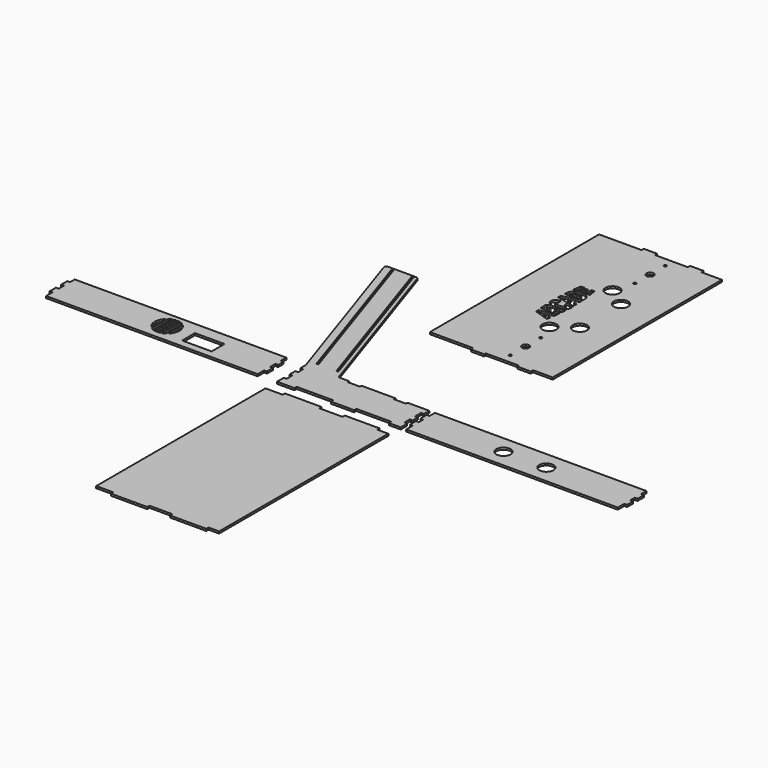
from build123d import *

# Parameters (mm, degrees)
F1_DEPTH = 4.45
F0_R     = 3
F0_R_2   = 8.087272744
F0_R_3   = 16.129
F0_W     = 66.7005181313
F0_H     = 36.3053381443


# Not quite as in the source:
# - ends of sketch curves that miss each other by under 0.0002 mm in the source are joined
# - a feature names something its author has since deleted; it is built from what else it names


with BuildPart() as f1:
    # F0 (on Top) → F1 (new body)
    with BuildSketch(Plane.XY):
        with BuildLine():
            Line((-13.1345508408, -164.6919741164), (-133.2231766972, 195.5739079059))
            ThreePointArc((-133.2231766972, 195.5739079059), (-135.0430417624, 198.0489800139), (-137.9665931933, 198.9927690934))
            Line((-137.9665931933, 198.9927690934), (-188.0199429035, 198.9927690934))
            Line((-188.0199429035, 198.9927690934), (-201.6566259516, 198.9927690934))
            ThreePointArc((-201.6566259516, 198.9927690934), (-205.7128368721, 196.9163205243), (-206.4000424478, 192.4116302809))
            Line((-206.4000424478, 192.4116302809), (-83.9924133672, -174.8112615001))
            Line((-83.9924133672, -174.8112615001), (-80.8544035681, -184.2252910137))
            Line((-80.8544035681, -184.2252910137), (-80.3456279762, -184.2252910137))
            Line((-80.3456279762, -184.2252910137), (-80.3456279762, -185.5896489572))
            Line((-80.3456279762, -185.5896489572), (-80.3456279762, -185.7516178083))
            Line((-80.3456279762, -185.7516178083), (-80.3456279762, -200.8809216976))
            Line((-80.3456279762, -200.8809216976), (-74.0156279762, -200.8809216976))
            Line((-74.0156279762, -200.8809216976), (-74.0156279762, -215.4068326941))
            Line((-74.0156279762, -215.4068326941), (-80.3456279762, -215.4068326941))
            Line((-80.3456279762, -215.4068326941), (-80.3456279762, -231.2078326941))
            Line((-80.3456279762, -231.2078326941), (-74.0156279762, -231.2078326941))
            Line((-74.0156279762, -231.2078326941), (-74.0156279762, -247.7338326941))
            Line((-74.0156279762, -247.7338326941), (-75.8956279762, -247.7338326941))
            Line((-75.8956279762, -247.7338326941), (-80.3456279762, -247.7338326941))
            Line((-80.3456279762, -247.7338326941), (-80.3456279762, -248.4956532717))
            Line((-80.3456279762, -248.4956532717), (-80.3456279762, -248.7336844206))
            Line((-80.3456279762, -248.7336844206), (-80.3456279762, -266.7746841908))
            Line((-80.3456279762, -266.7746841908), (-40.9429369935, -266.7746841908))
            Line((-40.9429369935, -266.7746841908), (-40.9429369935, -260.4446841907))
            Line((-40.9429369935, -260.4446841907), (41.3429330065, -260.4446841907))
            Line((41.3429330065, -260.4446841907), (41.3429330065, -266.7746841907))
            Line((41.3429330065, -266.7746841907), (93.9730530065, -266.7746841908))
            Line((93.9730530065, -266.7746841908), (93.9730530065, -260.4446841907))
            Line((93.9730530065, -260.4446841907), (172.7589230065, -260.4446841907))
            Line((172.7589230065, -260.4446841907), (172.7589230065, -266.7746841907))
            Line((172.7589230065, -266.7746841907), (199.3356065321, -266.7746841908))
            Line((199.3356065321, -266.7746841908), (199.3356065321, -248.4956532717))
            Line((199.3356065321, -248.4956532717), (193.0056065321, -248.4956532717))
            Line((193.0056065321, -248.4956532717), (193.0056065321, -232.9698022752))
            Line((193.0056065321, -232.9698022752), (199.3356065321, -232.9698022752))
            Line((199.3356065321, -232.9698022752), (199.3356065321, -218.5687422752))
            Line((199.3356065321, -218.5687422752), (193.0056065321, -218.5687422752))
            Line((193.0056065321, -218.5687422752), (193.0056065321, -201.0428905487))
            Line((193.0056065321, -201.0428905487), (199.3356065321, -201.0428905487))
            Line((199.3356065321, -201.0428905487), (199.3356065321, -185.7516178083))
            Line((199.3356065321, -185.7516178083), (149.9814315498, -185.7516178083))
            Line((149.9814315498, -185.7516178083), (149.9876286626, -190.2016178083))
            Line((149.9876286626, -190.2016178083), (122.5876286626, -190.2016178083))
            Line((122.5876286626, -190.2016178083), (122.5814315498, -185.7516178083))
            Line((122.5814315498, -185.7516178083), (45.8255372941, -185.7516178083))
            Line((45.8255372941, -185.7516178083), (45.8255372941, -190.2016178083))
            Line((45.8255372941, -190.2016178083), (18.4255372941, -190.2016178083))
            Line((18.4255372941, -190.2016178083), (17.9193401814, -185.7516178083))
            Line((17.9193401814, -185.7516178083), (-2.5108735826, -185.7516178083))
            ThreePointArc((-2.5108735826, -185.7516178083), (-5.4344250134, -184.8078287287), (-7.2542900787, -182.3327566208))
            Line((-7.2542900787, -182.3327566208), (-13.1345508408, -164.6919741164))
        make_face()
        Polygon((-68.8909804744, -169.5191176128), (-129.5292109794, 12.3955761507), (-190.322441274, 194.7752692889), (-185.872441274, 194.7752692889), (-125.1567108742, 12.6280758381), (-125.0792109794, 12.3955761507), (-64.4409804744, -169.5191176128), align=None, mode=Mode.SUBTRACT)
        Polygon((-145.372441274, 194.7752760296), (-140.922441274, 194.7752760296), (-19.4909804744, -169.5191108722), (-23.9409804744, -169.5191108722), (-84.6567108742, 12.6280825787), align=None, mode=Mode.SUBTRACT)
    extrude(amount=F1_DEPTH)


with BuildPart() as f1b:
    # F0 (on Top) → F1, piece 2 (new body)
    with BuildSketch(Plane.XY):
        Polygon((109.6645991251, 49.936733744), (109.6645991251, 43.606733744), (140.0583991251, 43.606733744), (140.0583991251, 48.056733744), (214.8266904935, 48.056733744), (214.8266904935, 43.606733744), (245.2266904935, 43.606733744), (245.2266904935, 49.936733744), (289.7008654758, 49.936733744), (289.7008654758, 528.386733744), (243.2266908545, 528.386733744), (243.2266908545, 534.716733744), (212.8266908545, 534.716733744), (212.8266908545, 528.386733744), (138.0584023733, 528.386733744), (138.0584023733, 534.716733744), (107.6646023733, 534.716733744), (107.6646023733, 528.386733744), (86.1305896078, 528.386733744), (11.8996296078, 528.386733744), (11.8996296078, 49.936733744), (86.1305896078, 49.936733744), align=None)
        with Locations((178.3758481905, 69.173247926)):
            Circle(F0_R, mode=Mode.SUBTRACT)
        with Locations((178.3758481905, 112.373247926)):
            Circle(F0_R_2, mode=Mode.SUBTRACT)
        with Locations((178.3758481905, 155.573247926)):
            Circle(F0_R, mode=Mode.SUBTRACT)
        with Locations((164.4027125835, 197.3344986652)):
            Circle(F0_R_3, mode=Mode.SUBTRACT)
        Polygon((144.38024237, 234.2502108202), (142.1130604967, 234.2502108202), (138.3344314918, 233.0626404271), (137.7946220263, 226.9088669107), (141.0334490165, 226.3150817141), (143.4625692591, 226.3150817141), (141.843155764, 218.1914640949), (140.1157833561, 218.9197583482), (134.9876381382, 220.3772260234), (123.0039752945, 224.2638251171), (109.6707962379, 228.5822598622), (108.9690484032, 235.0599175677), (128.5639636144, 238.406707196), (142.6528625115, 241.9694183752), (145.8329220252, 241.9694183752), align=None, mode=Mode.SUBTRACT)
        with BuildLine():
            add(Edge.make_bspline(
                [(128.5639636168, 260.5926792261), (126.6851334747, 261.6323850443), (125.1709058254, 262.4309195257), (123.2035912523, 262.8997626838)],
                knots=[0, 0, 0, 0, 0.1162972911, 0.1162972911, 0.1162972911, 0.1162972911], degree=3))
            add(Edge.make_bspline(
                [(131.0810425796, 258.8106178703), (130.4885197933, 259.5182474814), (129.4826550141, 260.0842943704), (128.5639636168, 260.5926792261)],
                knots=[0.9431341245, 0.9431341245, 0.9431341245, 0.9431341245, 1, 1, 1, 1], degree=3))
            Line((131.0810425796, 258.8106178703), (147.2951849037, 264.5332548154))
            Line((147.2951849037, 264.5332548154), (146.6391187302, 255.3441180101))
            Line((146.6391187302, 255.3441180101), (145.0819902192, 255.0326926987))
            Line((145.0819902192, 255.0326926987), (132.7204562794, 250.509393456))
            Line((132.7204562794, 250.509393456), (145.9027750667, 250.509393456))
            Line((145.9027750667, 250.509393456), (145.6217922195, 242.5632035718))
            Line((145.6217922195, 242.5632035718), (107.8536775567, 243.898710594))
            add(Edge.make_bspline(
                [(107.457601274, 243.9127161291), (107.5681389055, 243.8955344904), (107.7007268333, 243.8910975861), (107.8536775567, 243.898710594)],
                knots=[0.6431910445, 0.6431910445, 0.6431910445, 0.6431910445, 0.6525586544, 0.6525586544, 0.6525586544, 0.6525586544], degree=3))
            add(Edge.make_bspline(
                [(123.2035912523, 262.8997626838), (120.8214160248, 263.467473904), (114.6447375539, 263.6384105597), (104.4496833821, 259.1667517285), (108.5099601756, 247.3009629552), (106.515459915, 244.0591597631), (107.457601274, 243.9127161291)],
                knots=[0.1162972911, 0.1162972911, 0.1162972911, 0.1162972911, 0.2571189623, 0.4018084692, 0.5633484367, 0.6431910445, 0.6431910445, 0.6431910445, 0.6431910445], degree=3))
        make_face(mode=Mode.SUBTRACT)
        with BuildLine():
            add(Edge.make_bspline(
                [(118.4096939812, 278.2062657301), (118.008613675, 277.7544534713), (116.5254907196, 278.3846987718), (114.6860986223, 277.3704216428), (114.3121353636, 275.4818719009), (115.8822495107, 273.5639671058), (122.1543701521, 271.8085591307), (128.3372312156, 271.631565814), (134.6144229239, 272.2452065368), (138.281513843, 274.0041420395), (138.8901224926, 277.3280303811), (135.816879855, 277.8372704412), (132.3043819598, 278.6943910776), (132.8801296382, 279.7199041248), (133.0335295094, 286.4615207561), (131.517785638, 288.8097379759), (143.3081485383, 285.6706131454), (143.2876661042, 285.1920333687), (149.7203259126, 281.8270369122), (148.695702836, 273.0090093242), (145.8257996198, 267.8254041605), (137.5916580466, 263.7489152162), (126.7832057192, 262.9795878345), (114.9700731672, 264.1210882589), (108.486783454, 268.147637912), (104.5049371001, 272.096645925), (104.3359645468, 276.9661032929), (105.5397960824, 282.3849948376), (111.6880120097, 286.3382367425), (116.9904636561, 287.4430295691), (118.7674772932, 287.8835911533), (118.4200692992, 285.1487585296), (119.1960011795, 279.0920315629), (118.4096939812, 278.2062657301)],
                knots=[0, 0, 0, 0, 0.020494547, 0.0414693591, 0.0607350939, 0.0828404788, 0.1209521426, 0.159932456, 0.1980232824, 0.2276772762, 0.2510011815, 0.2764947931, 0.3037065377, 0.3173900946, 0.3574312462, 0.3741991924, 0.4232910827, 0.4368372532, 0.4735096835, 0.516799885, 0.5533151147, 0.5976483724, 0.648419728, 0.7005614172, 0.7421530316, 0.776720808, 0.8090959926, 0.8438514827, 0.8845213381, 0.9201032118, 0.9362852602, 0.9598209895, 1, 1, 1, 1], degree=3))
        make_face(mode=Mode.SUBTRACT)
        Polygon((146.2362490544, 313.2235731122), (146.9237737307, 313.160742366), (146.9237737307, 304.04164336), (144.6443654547, 304.04164336), (140.3559751758, 303.0352617738), (140.3559751758, 296.2421939832), (145.2770911107, 294.9842183974), (147.5267268667, 294.9842183974), (147.5016705642, 285.6739075454), (105.6019298682, 295.4861174461), (105.6019298682, 302.4049817708), align=None, mode=Mode.SUBTRACT)
        with BuildLine():
            ThreePointArc((107.1513079057, 320.8409628955), (125.426885077, 335.327875154), (146.2362490544, 324.7999257532))
            Line((146.2362490544, 324.7999257532), (146.9237737307, 313.6994063047))
            Line((146.9237737307, 313.6994063047), (106.4939506302, 312.5978863922))
            Line((106.4939506302, 312.5978863922), (107.1513079057, 320.8409628955))
        make_face(mode=Mode.SUBTRACT)
        Polygon((130.0334616295, 350.7802296276), (131.2729376142, 342.1865778554), (135.6725178609, 342.8211362717), (134.1524355063, 353.3603145865), (141.6923932681, 353.3603145865), (143.9817920473, 337.2012575192), (108.2818875652, 334.854008616), (111.446634675, 352.6165901807), (119.4676615248, 353.1822159079), (117.2535054335, 341.9162227896), (122.8425063143, 341.9162227896), (122.8425063143, 350.7802296276), align=None, mode=Mode.SUBTRACT)
        with Locations((208.4719767734, 228.5822598622)):
            Circle(F0_R_3, mode=Mode.SUBTRACT)
        with Locations((208.4719767734, 344.6277944729)):
            Circle(F0_R_3, mode=Mode.SUBTRACT)
        with Locations((164.4027125835, 375.8755556698)):
            Circle(F0_R_3, mode=Mode.SUBTRACT)
        with Locations((178.3758481905, 421.2868064091)):
            Circle(F0_R, mode=Mode.SUBTRACT)
        with Locations((178.3758481905, 464.4868064091)):
            Circle(F0_R_2, mode=Mode.SUBTRACT)
        with Locations((178.3758481905, 507.6868064091)):
            Circle(F0_R, mode=Mode.SUBTRACT)
        with BuildLine():
            Line((128.5639636168, 260.5926792261), (130.7771585832, 258.7033647236))
            Line((130.7771585832, 258.7033647236), (131.0810425796, 258.8106178703))
            add(Edge.make_bspline(
                [(131.0810425796, 258.8106178703), (130.4885197933, 259.5182474814), (129.4826550141, 260.0842943704), (128.5639636168, 260.5926792261)],
                knots=[0.9431341245, 0.9431341245, 0.9431341245, 0.9431341245, 1, 1, 1, 1], degree=3))
        make_face()
    extrude(amount=F1_DEPTH)


with BuildPart() as f1c:
    # F0 (on Top) → F1, piece 3 (new body)
    with BuildSketch(Plane.XY):
        Polygon((121.6972161211, 253.4000544932), (120.1217256436, 254.4976013836), (118.3763080916, 254.3745182559), (117.2535054335, 254.0755802312), (116.3434170136, 253.4000544932), (115.9999452481, 250.6342387882), (121.6972161211, 250.4327792945), align=None)
    extrude(amount=F1_DEPTH)


with BuildPart() as f1d:
    # F0 (on Top) → F1, piece 4 (new body)
    with BuildSketch(Plane.XY):
        Polygon((125.6387986193, 230.2756949452), (129.8662058959, 228.9461760905), (129.8662058959, 231.1009175268), align=None)
    extrude(amount=F1_DEPTH)


with BuildPart() as f1e:
    # F0 (on Top) → F1, piece 5 (new body)
    with BuildSketch(Plane.XY):
        Polygon((130.8137707362, 300.8135954973), (125.054859365, 299.5041205671), (130.8137707362, 298.1946465683), align=None)
    extrude(amount=F1_DEPTH)


with BuildPart() as f1f:
    # F0 (on Top) → F1, piece 6 (new body)
    with BuildSketch(Plane.XY):
        with BuildLine():
            Line((117.2535054335, 321.2757527021), (135.9537251243, 321.2757527021))
            Line((135.9537251243, 321.2757527021), (135.6725178609, 323.917501339))
            ThreePointArc((135.6725178609, 323.917501339), (126.3572301292, 327.5379858027), (117.2535054335, 323.4143114772))
            Line((117.2535054335, 323.4143114772), (117.2535054335, 321.2757527021))
        make_face()
    extrude(amount=F1_DEPTH)


with BuildPart() as f1g:
    # F0 (on Top) → F1, piece 7 (new body)
    with BuildSketch(Plane.XY):
        Polygon((690.2961595345, -185.7516178083), (211.8461595345, -185.7516178083), (211.8461595345, -201.0428905487), (205.5161595345, -201.0428905487), (205.5161595345, -218.5687422752), (211.8461595345, -218.5687422752), (211.8461595345, -226.2631509995), (211.8461595345, -230.9697422752), (205.5161595345, -230.9698015451), (205.5161595345, -248.4956532717), (211.8461595345, -248.4956532717), (211.8461595345, -266.7746841908), (690.2961595345, -266.7746841908), (690.2961595345, -248.4956532717), (696.6261595345, -248.4956532717), (696.6261595345, -230.9698015451), (690.2961595345, -230.9698015451), (690.2961595345, -218.5687422752), (696.6261595345, -218.5687422752), (696.6261595345, -201.0428905487), (690.2961595345, -201.0428905487), align=None)
        with Locations((399.4349042225, -226.2631509995)):
            Circle(F0_R_3, mode=Mode.SUBTRACT)
        with Locations((496.3774148464, -226.2631509995)):
            Circle(F0_R_3, mode=Mode.SUBTRACT)
    extrude(amount=F1_DEPTH)


with BuildPart() as f1h:
    # F0 (on Top) → F1, piece 8 (new body)
    with BuildSketch(Plane.XY):
        Polygon((-125.0792125037, -184.645057578), (-603.5792125037, -184.645057578), (-603.5792125037, -197.9363295884), (-609.9092125037, -197.9363295884), (-609.9092125037, -215.4621813149), (-603.5792125037, -215.4621813149), (-603.5792125037, -229.8632413149), (-609.9092125037, -229.8632413149), (-609.9092125037, -247.3890930414), (-603.5792125037, -247.3890930414), (-603.5792125037, -265.6681239605), (-125.0792125037, -265.6681239605), (-125.0792125037, -247.3890930414), (-118.7492125037, -247.3890930414), (-118.7492125037, -230.8632430414), (-125.0792125037, -230.8632430414), (-125.0792125037, -229.8632413149), (-125.0792125037, -215.4621813149), (-118.7492125037, -215.4621813149), (-118.7492125037, -200.9363313149), (-125.0792125037, -200.9363313149), align=None)
        with BuildLine():
            Line((-383.3327464205, -202.27664633), (-383.3327464205, -243.0487762998))
            ThreePointArc((-383.3327464205, -243.0487762998), (-392.1990159996, -222.6627113149), (-383.3327464205, -202.27664633))
        make_face(mode=Mode.SUBTRACT)
        with BuildLine():
            Line((-373.5705486876, -196.36967702), (-373.5705486876, -248.9557456098))
            ThreePointArc((-373.5705486876, -248.9557456098), (-377.1578306316, -247.4044271775), (-380.4928235156, -245.366535353))
            Line((-380.4928235156, -245.366535353), (-380.4928235156, -199.9588872768))
            ThreePointArc((-380.4928235156, -199.9588872768), (-377.4663403703, -197.3259929182), (-373.5705486876, -196.36967702))
        make_face(mode=Mode.SUBTRACT)
        with BuildLine():
            Line((-365.7607905013, -194.8296997759), (-365.7607905013, -250.4957228539))
            ThreePointArc((-365.7607905013, -250.4957228539), (-368.261689351, -250.253680358), (-370.7306257826, -249.787383754))
            Line((-370.7306257826, -249.787383754), (-370.7306257826, -195.5380388758))
            ThreePointArc((-370.7306257826, -195.5380388758), (-368.261689351, -195.0717422717), (-365.7607905013, -194.8296997759))
        make_face(mode=Mode.SUBTRACT)
        with BuildLine():
            ThreePointArc((-362.8976345062, -194.8296997759), (-360.3967356565, -195.0717422717), (-357.9277992249, -195.5380388758))
            Line((-357.9277992249, -195.5380388758), (-357.9277992249, -249.787383754))
            ThreePointArc((-357.9277992249, -249.787383754), (-360.3967356565, -250.253680358), (-362.8976345062, -250.4957228539))
            Line((-362.8976345062, -250.4957228539), (-362.8976345062, -194.8296997759))
        make_face(mode=Mode.SUBTRACT)
        with BuildLine():
            ThreePointArc((-348.1656014919, -245.366535353), (-351.5005943759, -247.4044271775), (-355.0878763199, -248.9557456098))
            Line((-355.0878763199, -248.9557456098), (-355.0878763199, -196.36967702))
            ThreePointArc((-355.0878763199, -196.36967702), (-351.5005943759, -197.9209954523), (-348.1656014919, -199.9588872768))
            Line((-348.1656014919, -199.9588872768), (-348.1656014919, -245.366535353))
        make_face(mode=Mode.SUBTRACT)
        with BuildLine():
            Line((-345.325678587, -243.0487762998), (-345.325678587, -202.27664633))
            ThreePointArc((-345.325678587, -202.27664633), (-336.4594090079, -222.6627113149), (-345.325678587, -243.0487762998))
        make_face(mode=Mode.SUBTRACT)
        with Locations((-276.2150764465, -230.4605394602)):
            Rectangle(F0_W, F0_H, mode=Mode.SUBTRACT)
    extrude(amount=F1_DEPTH)


with BuildPart() as f1i:
    # F0 (on Top) → F1, piece 9 (new body)
    with BuildSketch(Plane.XY):
        Polygon((-41.142935, -299.4968593121), (-80.3456306458, -299.4968593121), (-80.3456306458, -773.4968593121), (-80.3456306458, -777.9468593121), (-42.1429352306, -777.9468593121), (-42.1429352306, -784.2768593121), (40.1429347694, -784.2768593121), (40.1429347694, -777.9468593121), (91.3730523146, -777.9468593121), (91.3730523146, -784.2768593121), (173.6589223146, -784.2768593121), (173.6589223146, -777.9468593121), (197.4556038625, -777.9468593121), (197.4556038625, -299.4968593121), (175.6589227759, -299.4968593121), (172.758925, -299.4968593121), (172.758925, -293.1668593121), (93.973055, -293.1668593121), (93.973055, -299.4968593121), (41.142935, -299.4968593121), (41.142935, -293.1668593121), (-41.142935, -293.1668593121), align=None)
    extrude(amount=F1_DEPTH)


solid = Compound([f1.part, f1b.part, f1c.part, f1d.part, f1e.part, f1f.part, f1g.part, f1h.part, f1i.part])
